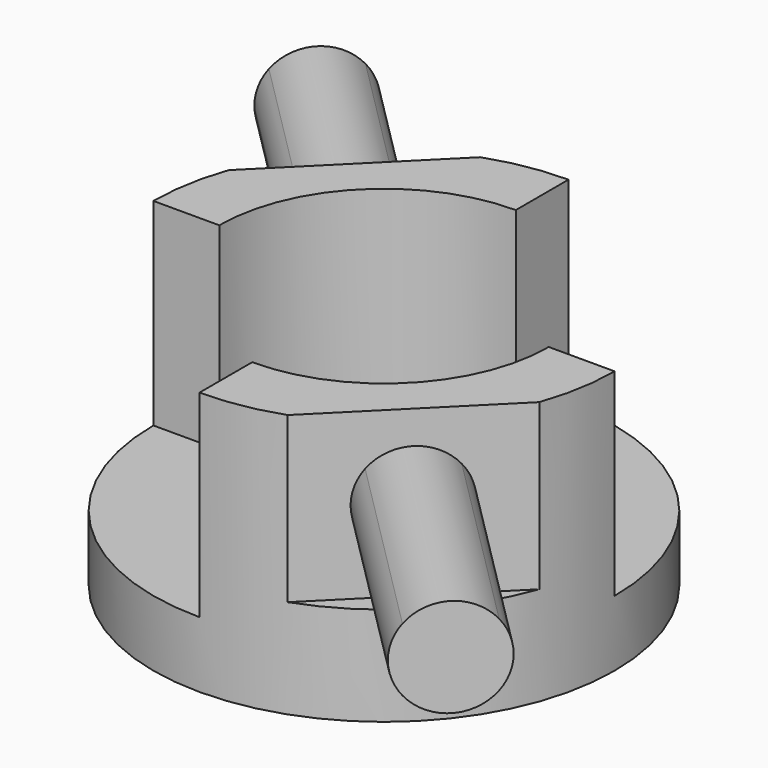
from build123d import *
from build123d import SkipClean  # not in build123d's __all__

# Parameters (mm, degrees)
F0_R     = 2
F1_DEPTH = 2
F3_DEPTH = 1
F5_DEPTH = 5
F8_DEPTH = 8
F9_DEPTH = 8


with BuildPart() as f1:
    # F0 (on Top) → F1 (new body)
    with BuildSketch(Plane.XY):
        with BuildLine():
            ThreePointArc((-5, 0), (-3.5355339059, 3.5355339059), (0, 5))
            Line((0, 5), (0, 7))
            ThreePointArc((0, 7), (-4.9497474683, 4.9497474683), (-7, 0))
            Line((-7, 0), (-5, 0))
        make_face()
        with BuildLine():
            ThreePointArc((0, 5), (3.5355339059, 3.5355339059), (5, 0))
            Line((5, 0), (7, 0))
            ThreePointArc((7, 0), (4.9497474683, 4.9497474683), (0, 7))
            Line((0, 7), (0, 5))
        make_face()
        with BuildLine():
            Line((7, 0), (5, 0))
            ThreePointArc((5, 0), (3.5355339059, -3.5355339059), (0, -5))
            Line((0, -5), (0, -7))
            ThreePointArc((0, -7), (4.9497474683, -4.9497474683), (7, 0))
        make_face()
        with BuildLine():
            Line((0, -7), (0, -5))
            ThreePointArc((0, -5), (-3.5355339059, -3.5355339059), (-5, 0))
            Line((-5, 0), (-7, 0))
            ThreePointArc((-7, 0), (-4.9497474683, -4.9497474683), (0, -7))
        make_face()
        with BuildLine():
            ThreePointArc((0, -5), (3.5355339059, -3.5355339059), (5, 0))
            ThreePointArc((5, 0), (3.5355339059, 3.5355339059), (0, 5))
            ThreePointArc((0, 5), (-3.5355339059, 3.5355339059), (-5, 0))
            ThreePointArc((-5, 0), (-3.5355339059, -3.5355339059), (0, -5))
        make_face()
        Circle(F0_R, mode=Mode.SUBTRACT)
    extrude(amount=F1_DEPTH)

    # F2 (on face) → F3 (join)
    with BuildSketch(Plane.XY.offset(2)):
        with BuildLine():
            ThreePointArc((-5, 0), (-3.5355339059, 3.5355339059), (0, 5))
            Line((0, 5), (0, 7))
            ThreePointArc((0, 7), (-1.1928549598, 6.8976153158), (-2.3508156114, 6.5934562986))
            Line((-2.3508156114, 6.5934562986), (-6.5934562986, 2.3508156114))
            ThreePointArc((-6.5934562986, 2.3508156114), (-6.8976153158, 1.1928549598), (-7, 0))
            Line((-7, 0), (-5, 0))
        make_face()
        with BuildLine():
            Line((-6.5934562986, 2.3508156114), (-2.3508156114, 6.5934562986))
            ThreePointArc((-2.3508156114, 6.5934562986), (-4.9497474683, 4.9497474683), (-6.5934562986, 2.3508156114))
        make_face()
        with BuildLine():
            ThreePointArc((2.3508156114, -6.5934562986), (4.9497474683, -4.9497474683), (6.5934562986, -2.3508156114))
            Line((6.5934562986, -2.3508156114), (2.3508156114, -6.5934562986))
        make_face()
        with BuildLine():
            Line((7, 0), (5, 0))
            ThreePointArc((5, 0), (3.5355339059, -3.5355339059), (0, -5))
            Line((0, -5), (0, -7))
            ThreePointArc((0, -7), (1.1928549598, -6.8976153158), (2.3508156114, -6.5934562986))
            Line((2.3508156114, -6.5934562986), (6.5934562986, -2.3508156114))
            ThreePointArc((6.5934562986, -2.3508156114), (6.8976153158, -1.1928549598), (7, 0))
        make_face()
    with SkipClean():  # cleaning this boolean's faces spoils the solid; the shape is the same uncleaned
        extrude(amount=F3_DEPTH)

    # F4 (on face) → F5 (join)
    with BuildSketch(Plane.XY.offset(3)):
        with BuildLine():
            ThreePointArc((-5, 0), (-3.5355339059, 3.5355339059), (0, 5))
            Line((0, 5), (0, 7))
            ThreePointArc((0, 7), (-1.1928549598, 6.8976153158), (-2.3508156114, 6.5934562986))
            Line((-2.3508156114, 6.5934562986), (-6.5934562986, 2.3508156114))
            ThreePointArc((-6.5934562986, 2.3508156114), (-6.8976153158, 1.1928549598), (-7, 0))
            Line((-7, 0), (-5, 0))
        make_face()
        with BuildLine():
            Line((7, 0), (5, 0))
            ThreePointArc((5, 0), (3.5355339059, -3.5355339059), (0, -5))
            Line((0, -5), (0, -7))
            ThreePointArc((0, -7), (1.1928549598, -6.8976153158), (2.3508156114, -6.5934562986))
            Line((2.3508156114, -6.5934562986), (6.5934562986, -2.3508156114))
            ThreePointArc((6.5934562986, -2.3508156114), (6.8976153158, -1.1928549598), (7, 0))
        make_face()
    extrude(amount=F5_DEPTH)

    # F7 (on face) → F8 (join)
    with BuildSketch(Plane(origin=(4.472135955, -4.472135955, 0), x_dir=(0.7071067812, 0.7071067812, 0), z_dir=(0.7071067812, -0.7071067812, 0))):
        with BuildLine():
            Line((1.1523319194, 6.4602765995), (0, 5.5))
            Line((0, 5.5), (1.1523319194, 4.5397234005))
            ThreePointArc((1.1523319194, 4.5397234005), (1.4104073665, 4.9893621044), (1.5, 5.5))
            ThreePointArc((1.5, 5.5), (1.4104073665, 6.0106378956), (1.1523319194, 6.4602765995))
        make_face()
        with BuildLine():
            Line((0, 5.5), (-1.1523319194, 6.4602765995))
            ThreePointArc((-1.1523319194, 6.4602765995), (-1.5, 5.5), (-1.1523319194, 4.5397234005))
            Line((-1.1523319194, 4.5397234005), (0, 5.5))
        make_face()
        with BuildLine():
            ThreePointArc((1.1523319194, 6.4602765995), (0, 7), (-1.1523319194, 6.4602765995))
            Line((-1.1523319194, 6.4602765995), (0, 5.5))
            Line((0, 5.5), (1.1523319194, 6.4602765995))
        make_face()
        with BuildLine():
            Line((1.1523319194, 4.5397234005), (0, 5.5))
            Line((0, 5.5), (-1.1523319194, 4.5397234005))
            ThreePointArc((-1.1523319194, 4.5397234005), (0, 4), (1.1523319194, 4.5397234005))
        make_face()
    extrude(amount=F8_DEPTH)

    # F6 (on face) → F9 (join)
    with BuildSketch(Plane(origin=(-4.472135955, 4.472135955, 0), x_dir=(-0.7071067812, -0.7071067812, 0), z_dir=(-0.7071067812, 0.7071067812, 0))):
        with BuildLine():
            ThreePointArc((1.1523319194, 6.4602765995), (0, 7), (-1.1523319194, 6.4602765995))
            Line((-1.1523319194, 6.4602765995), (0, 5.5))
            Line((0, 5.5), (1.1523319194, 6.4602765995))
        make_face()
        with BuildLine():
            Line((1.1523319194, 6.4602765995), (0, 5.5))
            Line((0, 5.5), (1.1523319194, 4.5397234005))
            ThreePointArc((1.1523319194, 4.5397234005), (1.4104073665, 4.9893621044), (1.5, 5.5))
            ThreePointArc((1.5, 5.5), (1.4104073665, 6.0106378956), (1.1523319194, 6.4602765995))
        make_face()
        with BuildLine():
            Line((1.1523319194, 4.5397234005), (0, 5.5))
            Line((0, 5.5), (-1.1523319194, 4.5397234005))
            ThreePointArc((-1.1523319194, 4.5397234005), (0, 4), (1.1523319194, 4.5397234005))
        make_face()
        with BuildLine():
            Line((0, 5.5), (-1.1523319194, 6.4602765995))
            ThreePointArc((-1.1523319194, 6.4602765995), (-1.5, 5.5), (-1.1523319194, 4.5397234005))
            Line((-1.1523319194, 4.5397234005), (0, 5.5))
        make_face()
    extrude(amount=F9_DEPTH)


solid = f1.part
